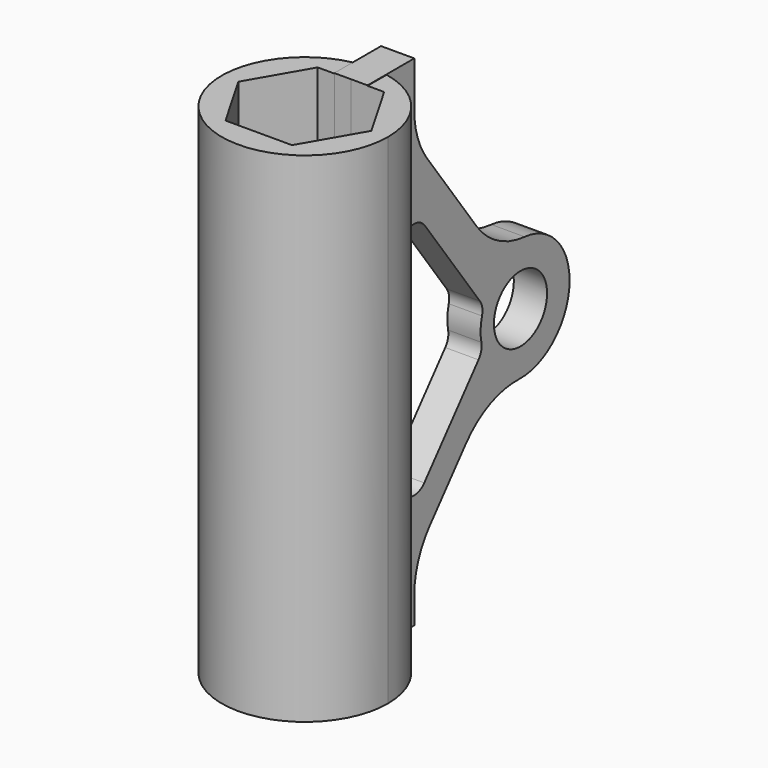
from build123d import *

# Parameters (mm, degrees)
F0_R     = 2
F1_DEPTH = 2
F3_DEPTH = 30


# Not quite as in the source:
# - ends of sketch curves that miss each other by under 0.0002 mm in the source are joined
# - a feature names something its author has since deleted; it is built from what else it names


with BuildPart() as f1:
    # F0 (on Right) → F1 (new body)
    with BuildSketch(Plane.YZ):
        with BuildLine():
            Line((-34.5930008724, 26.4829086736), (-38.1068567038, 26.4829086736))
            Line((-38.1068567038, 26.4829086736), (-38.1068567038, -3.5426183596))
            Line((-38.1068567038, -3.5426183596), (-34.5929991737, -3.5426183596))
            Line((-34.5929991737, -3.5426183596), (-34.5929991737, -1.9446051591))
            ThreePointArc((-34.5929991737, -1.9446051591), (-34.2912179318, -0.233833257), (-33.4223029733, 1.2704270974))
            Line((-33.4223029733, 1.2704270974), (-31.3919489583, 3.6887052743))
            Line((-31.3919489583, 3.6887052743), (-30.7011796085, 4.5114546232))
            ThreePointArc((-30.7011796085, 4.5114546232), (-28.9149664525, 5.8599495795), (-26.7193999751, 6.2940969379))
            ThreePointArc((-26.7193999751, 6.2940969379), (-22.9223984991, 9.7713294978), (-26.2963942816, 13.660354947))
            ThreePointArc((-26.2963942816, 13.660354947), (-28.3284558204, 14.2855279257), (-29.9170611144, 15.6984853104))
            Line((-29.9170611144, 15.6984853104), (-33.634288291, 20.8009439295))
            ThreePointArc((-33.634288291, 20.8009439295), (-34.3472851032, 22.1969357772), (-34.5930008724, 23.7450899858))
            Line((-34.5930008724, 23.7450899858), (-34.5930008724, 26.4829086736))
        make_face()
        with BuildLine():
            ThreePointArc((-29.6578618205, 11.6234470561), (-29.4825953492, 11.2153956919), (-29.5013036541, 10.771690552))
            ThreePointArc((-29.5013036541, 10.771690552), (-29.6050814327, 10.0861001216), (-29.5486860291, 9.3949969281))
            ThreePointArc((-29.5486860291, 9.3949969281), (-29.5605283151, 8.9510554769), (-29.7634350443, 8.5560198949))
            Line((-29.7634350443, 8.5560198949), (-33.8409951472, 3.699391672))
            ThreePointArc((-33.8409951472, 3.699391672), (-34.9490102875, 3.4027543717), (-35.6068559071, 4.3423981233))
            Line((-35.6068559071, 4.3423981233), (-35.6068559071, 16.7184074453))
            ThreePointArc((-35.6068559071, 16.7184074453), (-34.9164867488, 17.6692642914), (-33.7985984234, 17.3072366565))
            Line((-33.7985984234, 17.3072366565), (-29.6578618205, 11.6234470561))
        make_face(mode=Mode.SUBTRACT)
        with Locations((-26.6068567038, 9.9829086736)):
            Circle(F0_R, mode=Mode.SUBTRACT)
    extrude(amount=F1_DEPTH)

    # F2 (on face) → F3 (join)
    with BuildSketch(Plane(origin=(0, 0, -3.5426183596), x_dir=(1, 0, 0), z_dir=(0, 0, -1))):
        with BuildLine():
            Line((-1.0014715791, 45.0346349695), (2.9985283307, 45.035484586))
            Line((2.9985283307, 45.035484586), (4.9992640751, 41.5718078573))
            Line((4.9992640751, 41.5718078573), (2.9999999098, 38.107281512))
            Line((2.9999999098, 38.107281512), (0.9999999926, 38.1068567038))
            Line((0.9999999926, 38.1068567038), (2, 38.1068567038))
            Line((2, 38.1068567038), (2, 36.6721290144))
            ThreePointArc((2, 36.6721290144), (4.8724849939, 38.4089714581), (5.9992641654, 41.5709582407))
            ThreePointArc((5.9992641654, 41.5709582407), (-2.1633043456, 45.4437040901), (0, 36.6718286111))
            Line((0, 36.6718286111), (0, 38.1066442996))
            Line((0, 38.1066442996), (-1, 38.1064318955))
            Line((-1, 38.1064318955), (-3.0007357444, 41.5701086242))
            Line((-3.0007357444, 41.5701086242), (-1.0014715791, 45.0346349695))
        make_face()
    extrude(amount=-F3_DEPTH)


solid = f1.part
